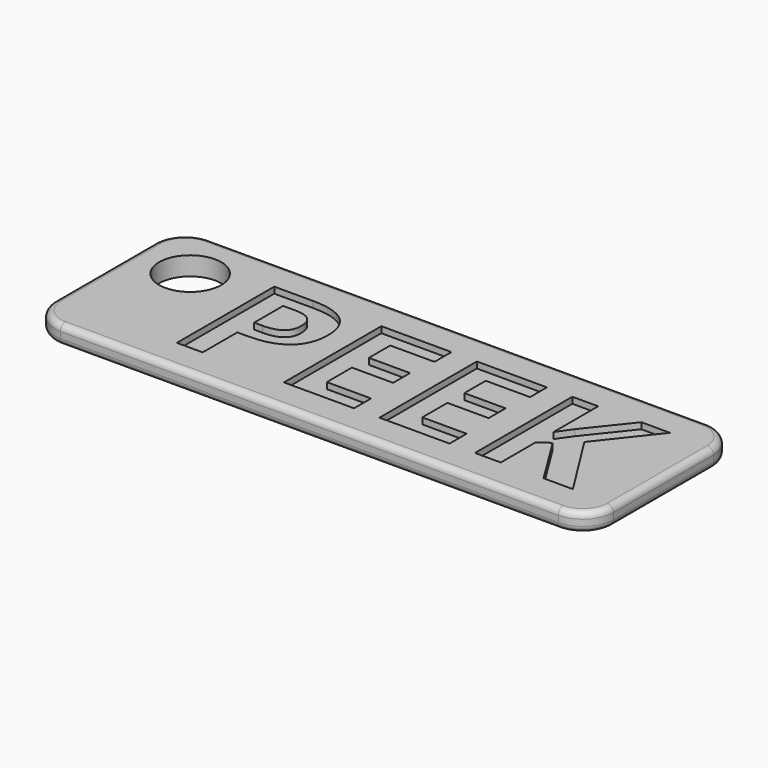
from build123d import *

# Parameters (mm, degrees)
F0_W         = 90
F0_H         = 30
F1_DEPTH     = 3
F2_R         = 1
F3_T1_DEPTH  = 3
F3_T4_ANGLE  = 90
F3_T6_ANGLE  = 90
F3_T8_ANGLE  = 90
F3_T10_ANGLE = 90
F3_T12_ANGLE = 90
F3_T14_ANGLE = 90
F3_T16_ANGLE = 90
F3_T18_ANGLE = 90
F4_R         = 5
F5_DEPTH     = 3
F6_TEXT_SIZE = 27.4539490285
F7_DEPTH     = 1


# Not quite as in the source:
# - a fillet or chamfer that OpenCascade refuses, or shapes differently, is made with other operations: its cross-section is extruded or revolved along the edge and cut away or added
# - Text() gives the source's letters only with a copy of the font that has no kerning and outlines rounded to 1/6400 em; it was checked with that copy


with BuildPart() as f1:
    # F0 (on Top) → F1 (new body)
    with BuildSketch(Plane.XY):
        Rectangle(F0_W, F0_H)
    extrude(amount=F1_DEPTH)

    # F2
    f2_edges = [f1.edges().sort_by_distance(p)[0] for p in [
        (0, 15, 3),
        (-45, 0, 3),
        (0, -15, 3),
        (45, 0, 3),
        (0, 15, 0),
        (-45, 0, 0),
        (0, -15, 0),
        (45, 0, 0),
    ]]
    fillet(f2_edges, radius=F2_R)

    # F3: fillet of radius 5 on 4 edges, made by hand

    # F3_s2 → F3_t1 (cut)
    with BuildSketch(Plane.XY):
        with BuildLine():
            ThreePointArc((45.0004, -9.9990343146), (43.5355339059, -13.5355339059), (39.9990343146, -15.0004))
            Line((39.9990343146, -15.0004), (39.9990343146, -15.5005365685))
            ThreePointArc((39.9990343146, -15.5005365685), (42.4995171573, -15.5001365685), (45, -15.5001365685))
            Line((45, -15.5001365685), (45.5001365685, -15))
            ThreePointArc((45.5001365685, -15), (45.5001365685, -12.4995171573), (45.5005365685, -9.9990343146))
            Line((45.5005365685, -9.9990343146), (45.0004, -9.9990343146))
        make_face()
        with BuildLine():
            ThreePointArc((39.9990343146, 15.0004), (43.5355339059, 13.5355339059), (45.0004, 9.9990343146))
            Line((45.0004, 9.9990343146), (45.5005365685, 9.9990343146))
            ThreePointArc((45.5005365685, 9.9990343146), (45.5001365685, 12.4995171573), (45.5001365685, 15))
            Line((45.5001365685, 15), (45, 15.5001365685))
            ThreePointArc((45, 15.5001365685), (42.4995171573, 15.5001365685), (39.9990343146, 15.5005365685))
            Line((39.9990343146, 15.5005365685), (39.9990343146, 15.0004))
        make_face()
        with BuildLine():
            ThreePointArc((-39.9990343146, 15.0004), (-43.5355339059, 13.5355339059), (-45.0004, 9.9990343146))
            Line((-45.0004, 9.9990343146), (-45.5005365685, 9.9990343146))
            ThreePointArc((-45.5005365685, 9.9990343146), (-45.5001365685, 12.4995171573), (-45.5001365685, 15))
            Line((-45.5001365685, 15), (-45, 15.5001365685))
            ThreePointArc((-45, 15.5001365685), (-42.4995171573, 15.5001365685), (-39.9990343146, 15.5005365685))
            Line((-39.9990343146, 15.5005365685), (-39.9990343146, 15.0004))
        make_face()
        with BuildLine():
            ThreePointArc((-45.0004, -9.9990343146), (-43.5355339059, -13.5355339059), (-39.9990343146, -15.0004))
            Line((-39.9990343146, -15.0004), (-39.9990343146, -15.5005365685))
            ThreePointArc((-39.9990343146, -15.5005365685), (-42.4995171573, -15.5001365685), (-45, -15.5001365685))
            Line((-45, -15.5001365685), (-45.5001365685, -15))
            ThreePointArc((-45.5001365685, -15), (-45.5001365685, -12.4995171573), (-45.5005365685, -9.9990343146))
            Line((-45.5005365685, -9.9990343146), (-45.0004, -9.9990343146))
        make_face()
    extrude(amount=F3_T1_DEPTH, mode=Mode.SUBTRACT)

    # F3_s3 → F3_t4 (revolve, cut)
    with BuildSketch(Plane.YZ.offset(-39.9990343146)):
        with BuildLine():
            ThreePointArc((-14.0004, 0), (-14.7075067812, 0.2928932188), (-15.0004, 1))
            Line((-15.0004, 1), (-15.0004, 0))
            Line((-15.0004, 0), (-14.0004, 0))
        make_face()
    revolve(axis=Axis((-39.9990343146, -9.9990343146, 0), (0, 0, -1)), revolution_arc=F3_T4_ANGLE, mode=Mode.SUBTRACT)

    # F3_s5 → F3_t6 (revolve, cut)
    with BuildSketch(Plane.XZ.offset(9.9990343146)):
        with BuildLine():
            ThreePointArc((-44.0004, 3), (-44.7075067812, 2.7071067812), (-45.0004, 2))
            Line((-45.0004, 2), (-45.0004, 3))
            Line((-45.0004, 3), (-44.0004, 3))
        make_face()
    revolve(axis=Axis((-39.9990343146, -9.9990343146, 3), (0, 0, 1)), revolution_arc=F3_T6_ANGLE, mode=Mode.SUBTRACT)

    # F3_s7 → F3_t8 (revolve, cut)
    with BuildSketch(Plane.XZ.offset(-9.9990343146)):
        with BuildLine():
            ThreePointArc((-44.0004, 0), (-44.7075067812, 0.2928932188), (-45.0004, 1))
            Line((-45.0004, 1), (-45.0004, 0))
            Line((-45.0004, 0), (-44.0004, 0))
        make_face()
    revolve(axis=Axis((-39.9990343146, 9.9990343146, 0), (0, 0, -1)), revolution_arc=F3_T8_ANGLE, mode=Mode.SUBTRACT)

    # F3_s9 → F3_t10 (revolve, cut)
    with BuildSketch(Plane.YZ.offset(-39.9990343146)):
        with BuildLine():
            ThreePointArc((14.0004, 3), (14.7075067812, 2.7071067812), (15.0004, 2))
            Line((15.0004, 2), (15.0004, 3))
            Line((15.0004, 3), (14.0004, 3))
        make_face()
    revolve(axis=Axis((-39.9990343146, 9.9990343146, 3), (0, 0, 1)), revolution_arc=F3_T10_ANGLE, mode=Mode.SUBTRACT)

    # F3_s11 → F3_t12 (revolve, cut)
    with BuildSketch(Plane.YZ.offset(39.9990343146)):
        with BuildLine():
            ThreePointArc((14.0004, 0), (14.7075067812, 0.2928932188), (15.0004, 1))
            Line((15.0004, 1), (15.0004, 0))
            Line((15.0004, 0), (14.0004, 0))
        make_face()
    revolve(axis=Axis((39.9990343146, 9.9990343146, 0), (0, 0, -1)), revolution_arc=F3_T12_ANGLE, mode=Mode.SUBTRACT)

    # F3_s13 → F3_t14 (revolve, cut)
    with BuildSketch(Plane.XZ.offset(-9.9990343146)):
        with BuildLine():
            ThreePointArc((44.0004, 3), (44.7075067812, 2.7071067812), (45.0004, 2))
            Line((45.0004, 2), (45.0004, 3))
            Line((45.0004, 3), (44.0004, 3))
        make_face()
    revolve(axis=Axis((39.9990343146, 9.9990343146, 3), (0, 0, 1)), revolution_arc=F3_T14_ANGLE, mode=Mode.SUBTRACT)

    # F3_s15 → F3_t16 (revolve, cut)
    with BuildSketch(Plane.XZ.offset(9.9990343146)):
        with BuildLine():
            ThreePointArc((44.0004, 0), (44.7075067812, 0.2928932188), (45.0004, 1))
            Line((45.0004, 1), (45.0004, 0))
            Line((45.0004, 0), (44.0004, 0))
        make_face()
    revolve(axis=Axis((39.9990343146, -9.9990343146, 0), (0, 0, -1)), revolution_arc=F3_T16_ANGLE, mode=Mode.SUBTRACT)

    # F3_s17 → F3_t18 (revolve, cut)
    with BuildSketch(Plane.YZ.offset(39.9990343146)):
        with BuildLine():
            ThreePointArc((-14.0004, 3), (-14.7075067812, 2.7071067812), (-15.0004, 2))
            Line((-15.0004, 2), (-15.0004, 3))
            Line((-15.0004, 3), (-14.0004, 3))
        make_face()
    revolve(axis=Axis((39.9990343146, -9.9990343146, 3), (0, 0, 1)), revolution_arc=F3_T18_ANGLE, mode=Mode.SUBTRACT)

    # F4 (on face) → F5 (cut)
    with BuildSketch(Plane.XY.offset(3)):
        with Locations((-36, 6)):
            Circle(F4_R)
    extrude(amount=-F5_DEPTH, mode=Mode.SUBTRACT)

    # F6 (on face) → F7 (cut)
    with BuildSketch(Plane.XY.offset(3)):
        with Locations((-28, -9.7668433005)):
            Text('PEEK', F6_TEXT_SIZE, font='Open Sans', font_style=FontStyle.BOLD, text_align=(TextAlign.LEFT, TextAlign.BOTTOM))
    extrude(amount=-F7_DEPTH, mode=Mode.SUBTRACT)


solid = f1.part
